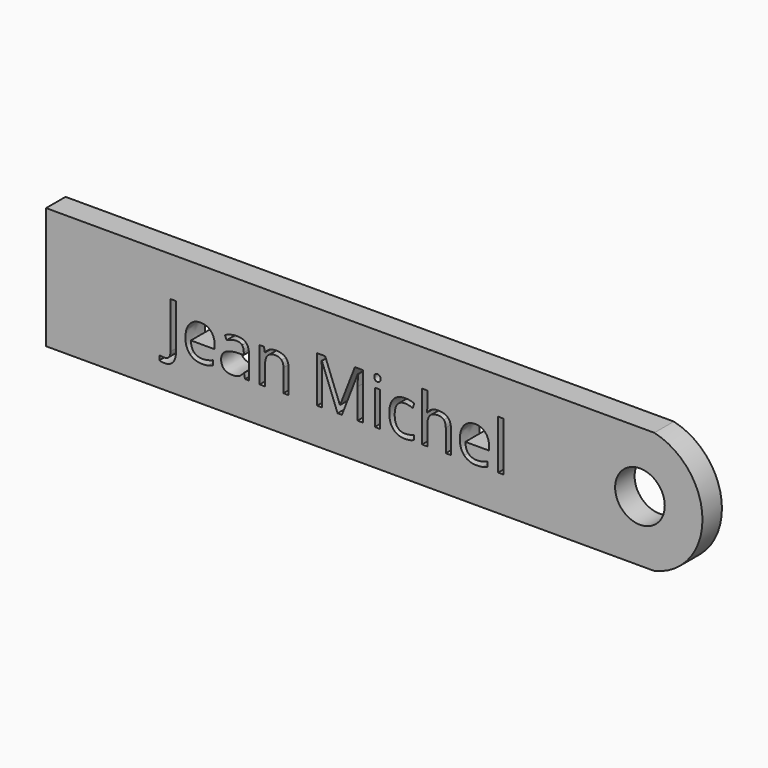
from build123d import *

# Parameters (mm, degrees)
F0_W     = 0.4318458111
F0_H     = 2.8498495239
F0_H_2   = 4.0463702874
F0_R     = 2.0408732003
F1_DEPTH = 2


with BuildPart() as f1:
    # F0 (on Front) → F1 (new body)
    with BuildSketch(Plane.XZ):
        with BuildLine():
            Line((30.7838568464, 24.9683012729), (-19.2161431536, 24.9683012729))
            Line((-19.2161431536, 24.9683012729), (-19.2161431536, 14.9683012729))
            Line((-19.2161431536, 14.9683012729), (30.7838568464, 14.9683012729))
            ThreePointArc((30.7838568464, 14.9683012729), (34.7379549914, 19.9683012729), (30.7838568464, 24.9683012729))
        make_face()
        with BuildLine():
            add(Edge.make_bspline(
                [(-8.7974733445, 17.1836813513), (-9.0470952006, 16.9120095646), (-9.5155522172, 16.9120095646)],
                knots=[0, 0, 0, 1, 1, 1], degree=2))
            add(Edge.make_bspline(
                [(-9.5155522172, 16.9120095646), (-9.7593495634, 16.9120095646), (-9.8999698756, 16.9819036843)],
                knots=[0, 0, 0, 1, 1, 1], degree=2))
            Line((-9.8999698756, 16.9819036843), (-9.8999698756, 17.358832687))
            add(Edge.make_bspline(
                [(-9.8999698756, 17.358832687), (-9.7152497021, 17.3072441701), (-9.5155522172, 17.3072441701)],
                knots=[0, 0, 0, 1, 1, 1], degree=2))
            add(Edge.make_bspline(
                [(-9.5155522172, 17.3072441701), (-9.2576096326, 17.3072441701), (-9.1236459031, 17.4632578302)],
                knots=[0, 0, 0, 1, 1, 1], degree=2))
            add(Edge.make_bspline(
                [(-9.1236459031, 17.4632578302), (-8.9896821737, 17.6192714902), (-8.9896821737, 17.9129932076)],
                knots=[0, 0, 0, 1, 1, 1], degree=2))
            Line((-8.9896821737, 17.9129932076), (-8.9896821737, 21.714734076))
            Line((-8.9896821737, 21.714734076), (-8.5478514884, 21.714734076))
            Line((-8.5478514884, 21.714734076), (-8.5478514884, 17.9496044131))
            add(Edge.make_bspline(
                [(-8.5478514884, 17.9496044131), (-8.5478514884, 17.455353138), (-8.7974733445, 17.1836813513)],
                knots=[0, 0, 0, 1, 1, 1], degree=2))
        make_face(mode=Mode.SUBTRACT)
        with BuildLine():
            add(Edge.make_bspline(
                [(-5.9076843237, 17.9038404062), (-6.1115421728, 17.8605726178), (-6.4002714531, 17.8605726178)],
                knots=[0, 0, 0, 1, 1, 1], degree=2))
            add(Edge.make_bspline(
                [(-6.4002714531, 17.8605726178), (-7.031814749, 17.8605726178), (-7.3975107682, 18.245822349)],
                knots=[0, 0, 0, 1, 1, 1], degree=2))
            add(Edge.make_bspline(
                [(-7.3975107682, 18.245822349), (-7.7632067874, 18.6310720803), (-7.7632067874, 19.3142038932)],
                knots=[0, 0, 0, 1, 1, 1], degree=2))
            add(Edge.make_bspline(
                [(-7.7632067874, 19.3142038932), (-7.7632067874, 20.0039922889), (-7.4237210631, 20.409627805)],
                knots=[0, 0, 0, 1, 1, 1], degree=2))
            add(Edge.make_bspline(
                [(-7.4237210631, 20.409627805), (-7.0842353388, 20.8152633212), (-6.5117692154, 20.8152633212)],
                knots=[0, 0, 0, 1, 1, 1], degree=2))
            add(Edge.make_bspline(
                [(-6.5117692154, 20.8152633212), (-5.9767463705, 20.8152633212), (-5.6647190504, 20.4628804677)],
                knots=[0, 0, 0, 1, 1, 1], degree=2))
            add(Edge.make_bspline(
                [(-5.6647190504, 20.4628804677), (-5.3526917303, 20.1104976141), (-5.3526917303, 19.5330390537)],
                knots=[0, 0, 0, 1, 1, 1], degree=2))
            Line((-5.3526917303, 19.5330390537), (-5.3526917303, 19.2601191577))
            Line((-5.3526917303, 19.2601191577), (-7.3155515921, 19.2601191577))
            add(Edge.make_bspline(
                [(-7.3155515921, 19.2601191577), (-7.3022384264, 18.7583792269), (-7.0617693717, 18.4983564601)],
                knots=[0, 0, 0, 1, 1, 1], degree=2))
            add(Edge.make_bspline(
                [(-7.0617693717, 18.4983564601), (-6.821300317, 18.2383336934), (-6.3844620688, 18.2383336934)],
                knots=[0, 0, 0, 1, 1, 1], degree=2))
            add(Edge.make_bspline(
                [(-6.3844620688, 18.2383336934), (-5.9243257807, 18.2383336934), (-5.4750064398, 18.4305425226)],
                knots=[0, 0, 0, 1, 1, 1], degree=2))
            Line((-5.4750064398, 18.4305425226), (-5.4750064398, 18.0452927913))
            add(Edge.make_bspline(
                [(-5.4750064398, 18.0452927913), (-5.7038264745, 17.9471081946), (-5.9076843237, 17.9038404062)],
                knots=[0, 0, 0, 1, 1, 1], degree=2))
        make_face(mode=Mode.SUBTRACT)
        with BuildLine():
            Line((-2.5436137762, 17.9129932076), (-2.8639618249, 17.9129932076))
            Line((-2.8639618249, 17.9129932076), (-2.9496653288, 18.3190447602))
            Line((-2.9496653288, 18.3190447602), (-2.9704671502, 18.3190447602))
            add(Edge.make_bspline(
                [(-2.9704671502, 18.3190447602), (-3.1834778007, 18.0511173013), (-3.395240342, 17.9558449595)],
                knots=[0, 0, 0, 1, 1, 1], degree=2))
            add(Edge.make_bspline(
                [(-3.395240342, 17.9558449595), (-3.6070028833, 17.8605726178), (-3.9248547134, 17.8605726178)],
                knots=[0, 0, 0, 1, 1, 1], degree=2))
            add(Edge.make_bspline(
                [(-3.9248547134, 17.8605726178), (-4.3483797959, 17.8605726178), (-4.5888488506, 18.0794077783)],
                knots=[0, 0, 0, 1, 1, 1], degree=2))
            add(Edge.make_bspline(
                [(-4.5888488506, 18.0794077783), (-4.8293179053, 18.2982429388), (-4.8293179053, 18.7009662)],
                knots=[0, 0, 0, 1, 1, 1], degree=2))
            add(Edge.make_bspline(
                [(-4.8293179053, 18.7009662), (-4.8293179053, 19.5638257493), (-3.4489090411, 19.605429392)],
                knots=[0, 0, 0, 1, 1, 1], degree=2))
            Line((-3.4489090411, 19.605429392), (-2.9654747131, 19.6212387762))
            Line((-2.9654747131, 19.6212387762), (-2.9654747131, 19.798470294))
            add(Edge.make_bspline(
                [(-2.9654747131, 19.798470294), (-2.9654747131, 20.133795654), (-3.1094233168, 20.293553642)],
                knots=[0, 0, 0, 1, 1, 1], degree=2))
            add(Edge.make_bspline(
                [(-3.1094233168, 20.293553642), (-3.2533719204, 20.4533116299), (-3.5712237505, 20.4533116299)],
                knots=[0, 0, 0, 1, 1, 1], degree=2))
            add(Edge.make_bspline(
                [(-3.5712237505, 20.4533116299), (-3.9273509319, 20.4533116299), (-4.3766702729, 20.2353085422)],
                knots=[0, 0, 0, 1, 1, 1], degree=2))
            Line((-4.3766702729, 20.2353085422), (-4.5098019295, 20.5656414651))
            add(Edge.make_bspline(
                [(-4.5098019295, 20.5656414651), (-4.2992874975, 20.6796354461), (-4.0484175321, 20.7445371286)],
                knots=[0, 0, 0, 1, 1, 1], degree=2))
            add(Edge.make_bspline(
                [(-4.0484175321, 20.7445371286), (-3.7975475667, 20.8094388112), (-3.5445974192, 20.8094388112)],
                knots=[0, 0, 0, 1, 1, 1], degree=2))
            add(Edge.make_bspline(
                [(-3.5445974192, 20.8094388112), (-3.0353688328, 20.8094388112), (-2.7894913045, 20.5835310315)],
                knots=[0, 0, 0, 1, 1, 1], degree=2))
            add(Edge.make_bspline(
                [(-2.7894913045, 20.5835310315), (-2.5436137762, 20.3576232517), (-2.5436137762, 19.8583795395)],
                knots=[0, 0, 0, 1, 1, 1], degree=2))
            Line((-2.5436137762, 19.8583795395), (-2.5436137762, 17.9129932076))
        make_face(mode=Mode.SUBTRACT)
        with BuildLine():
            Line((0.7272646116, 17.9129932076), (0.2954188005, 17.9129932076))
            Line((0.2954188005, 17.9129932076), (0.2954188005, 19.7568666513))
            add(Edge.make_bspline(
                [(0.2954188005, 19.7568666513), (0.2954188005, 20.1046731042), (0.1369089219, 20.2764961485)],
                knots=[0, 0, 0, 1, 1, 1], degree=2))
            add(Edge.make_bspline(
                [(0.1369089219, 20.2764961485), (-0.0216009567, 20.4483191927), (-0.3602546082, 20.4483191927)],
                knots=[0, 0, 0, 1, 1, 1], degree=2))
            add(Edge.make_bspline(
                [(-0.3602546082, 20.4483191927), (-0.8070777306, 20.4483191927), (-1.015095944, 20.2066020287)],
                knots=[0, 0, 0, 1, 1, 1], degree=2))
            add(Edge.make_bspline(
                [(-1.015095944, 20.2066020287), (-1.2231141575, 19.9648848647), (-1.2231141575, 19.4082281256)],
                knots=[0, 0, 0, 1, 1, 1], degree=2))
            Line((-1.2231141575, 19.4082281256), (-1.2231141575, 17.9129932076))
            Line((-1.2231141575, 17.9129932076), (-1.6549599685, 17.9129932076))
            Line((-1.6549599685, 17.9129932076), (-1.6549599685, 20.7628427314))
            Line((-1.6549599685, 20.7628427314), (-1.3038252243, 20.7628427314))
            Line((-1.3038252243, 20.7628427314), (-1.2339311046, 20.3726005631))
            Line((-1.2339311046, 20.3726005631), (-1.2131292832, 20.3726005631))
            add(Edge.make_bspline(
                [(-1.2131292832, 20.3726005631), (-1.0799976266, 20.583114995), (-0.8407766812, 20.6991891581)],
                knots=[0, 0, 0, 1, 1, 1], degree=2))
            add(Edge.make_bspline(
                [(-0.8407766812, 20.6991891581), (-0.6015557358, 20.8152633212), (-0.3078340184, 20.8152633212)],
                knots=[0, 0, 0, 1, 1, 1], degree=2))
            add(Edge.make_bspline(
                [(-0.3078340184, 20.8152633212), (0.207219078, 20.8152633212), (0.4672418448, 20.5668895744)],
                knots=[0, 0, 0, 1, 1, 1], degree=2))
            add(Edge.make_bspline(
                [(0.4672418448, 20.5668895744), (0.7272646116, 20.3185158276), (0.7272646116, 19.7718439627)],
                knots=[0, 0, 0, 1, 1, 1], degree=2))
            Line((0.7272646116, 19.7718439627), (0.7272646116, 17.9129932076))
        make_face(mode=Mode.SUBTRACT)
        with BuildLine():
            Line((5.1006395305, 17.9129932076), (4.7445123491, 17.9129932076))
            Line((4.7445123491, 17.9129932076), (3.4547994259, 21.282888265))
            Line((3.4547994259, 21.282888265), (3.4339976046, 21.282888265))
            add(Edge.make_bspline(
                [(3.4339976046, 21.282888265), (3.4706088102, 20.8826612224), (3.4706088102, 20.3309969204)],
                knots=[0, 0, 0, 1, 1, 1], degree=2))
            Line((3.4706088102, 20.3309969204), (3.4706088102, 17.9129932076))
            Line((3.4706088102, 17.9129932076), (3.062061039, 17.9129932076))
            Line((3.062061039, 17.9129932076), (3.062061039, 21.714734076))
            Line((3.062061039, 21.714734076), (3.7277193219, 21.714734076))
            Line((3.7277193219, 21.714734076), (4.9317287412, 18.5786514905))
            Line((4.9317287412, 18.5786514905), (4.9525305626, 18.5786514905))
            Line((4.9525305626, 18.5786514905), (6.1665248561, 21.714734076))
            Line((6.1665248561, 21.714734076), (6.8271907019, 21.714734076))
            Line((6.8271907019, 21.714734076), (6.8271907019, 17.9129932076))
            Line((6.8271907019, 17.9129932076), (6.3853600166, 17.9129932076))
            Line((6.3853600166, 17.9129932076), (6.3853600166, 20.3626156888))
            add(Edge.make_bspline(
                [(6.3853600166, 20.3626156888), (6.3853600166, 20.7836445528), (6.4219712222, 21.2778958279)],
                knots=[0, 0, 0, 1, 1, 1], degree=2))
            Line((6.4219712222, 21.2778958279), (6.4011694008, 21.2778958279))
            Line((6.4011694008, 21.2778958279), (5.1006395305, 17.9129932076))
        make_face(mode=Mode.SUBTRACT)
        with Locations((8.0207992105, 19.3379179695)):
            Rectangle(F0_W, F0_H, mode=Mode.SUBTRACT)
        with BuildLine():
            add(Edge.make_bspline(
                [(11.0108530102, 18.0095136586), (10.7254520214, 17.8605726178), (10.2911099918, 17.8605726178)],
                knots=[0, 0, 0, 1, 1, 1], degree=2))
            add(Edge.make_bspline(
                [(10.2911099918, 17.8605726178), (9.6720477886, 17.8605726178), (9.3325620643, 18.2416619848)],
                knots=[0, 0, 0, 1, 1, 1], degree=2))
            add(Edge.make_bspline(
                [(9.3325620643, 18.2416619848), (8.99307634, 18.6227513518), (8.99307634, 19.3200284031)],
                knots=[0, 0, 0, 1, 1, 1], degree=2))
            add(Edge.make_bspline(
                [(8.99307634, 19.3200284031), (8.99307634, 20.0347789845), (9.3379705379, 20.4250211528)],
                knots=[0, 0, 0, 1, 1, 1], degree=2))
            add(Edge.make_bspline(
                [(9.3379705379, 20.4250211528), (9.6828647357, 20.8152633212), (10.3194004688, 20.8152633212)],
                knots=[0, 0, 0, 1, 1, 1], degree=2))
            add(Edge.make_bspline(
                [(10.3194004688, 20.8152633212), (10.5249224636, 20.8152633212), (10.7304444585, 20.7707474235)],
                knots=[0, 0, 0, 1, 1, 1], degree=2))
            add(Edge.make_bspline(
                [(10.7304444585, 20.7707474235), (10.9359664534, 20.7262315259), (11.0524566529, 20.6663222804)],
                knots=[0, 0, 0, 1, 1, 1], degree=2))
            Line((11.0524566529, 20.6663222804), (10.9201570691, 20.3002102248))
            add(Edge.make_bspline(
                [(10.9201570691, 20.3002102248), (10.7770405383, 20.3576232517), (10.608129749, 20.3950665301)],
                knots=[0, 0, 0, 1, 1, 1], degree=2))
            add(Edge.make_bspline(
                [(10.608129749, 20.3950665301), (10.4392189597, 20.4325098085), (10.3094155945, 20.4325098085)],
                knots=[0, 0, 0, 1, 1, 1], degree=2))
            add(Edge.make_bspline(
                [(10.3094155945, 20.4325098085), (9.4407315353, 20.4325098085), (9.4407315353, 19.3250208403)],
                knots=[0, 0, 0, 1, 1, 1], degree=2))
            add(Edge.make_bspline(
                [(9.4407315353, 19.3250208403), (9.4407315353, 18.7999828696), (9.6524940766, 18.5191582815)],
                knots=[0, 0, 0, 1, 1, 1], degree=2))
            add(Edge.make_bspline(
                [(9.6524940766, 18.5191582815), (9.8642566178, 18.2383336934), (10.2802930447, 18.2383336934)],
                knots=[0, 0, 0, 1, 1, 1], degree=2))
            add(Edge.make_bspline(
                [(10.2802930447, 18.2383336934), (10.636420226, 18.2383336934), (11.0108530102, 18.3914350984)],
                knots=[0, 0, 0, 1, 1, 1], degree=2))
            Line((11.0108530102, 18.3914350984), (11.0108530102, 18.0095136586))
        make_face(mode=Mode.SUBTRACT)
        with BuildLine():
            Line((14.0695528203, 17.9129932076), (13.6377070093, 17.9129932076))
            Line((13.6377070093, 17.9129932076), (13.6377070093, 19.7568666513))
            add(Edge.make_bspline(
                [(13.6377070093, 19.7568666513), (13.6377070093, 20.1046731042), (13.4791971306, 20.2764961485)],
                knots=[0, 0, 0, 1, 1, 1], degree=2))
            add(Edge.make_bspline(
                [(13.4791971306, 20.2764961485), (13.320687252, 20.4483191927), (12.9820336006, 20.4483191927)],
                knots=[0, 0, 0, 1, 1, 1], degree=2))
            add(Edge.make_bspline(
                [(12.9820336006, 20.4483191927), (12.5327142596, 20.4483191927), (12.3259441554, 20.2036897738)],
                knots=[0, 0, 0, 1, 1, 1], degree=2))
            add(Edge.make_bspline(
                [(12.3259441554, 20.2036897738), (12.1191740513, 19.9590603548), (12.1191740513, 19.4032356885)],
                knots=[0, 0, 0, 1, 1, 1], degree=2))
            Line((12.1191740513, 19.4032356885), (12.1191740513, 17.9129932076))
            Line((12.1191740513, 17.9129932076), (11.6873282402, 17.9129932076))
            Line((11.6873282402, 17.9129932076), (11.6873282402, 21.959363495))
            Line((11.6873282402, 21.959363495), (12.1191740513, 21.959363495))
            Line((12.1191740513, 21.959363495), (12.1191740513, 20.7345522544))
            add(Edge.make_bspline(
                [(12.1191740513, 20.7345522544), (12.1191740513, 20.5132208753), (12.09837223, 20.3676081259)],
                knots=[0, 0, 0, 1, 1, 1], degree=2))
            Line((12.09837223, 20.3676081259), (12.1241664884, 20.3676081259))
            add(Edge.make_bspline(
                [(12.1241664884, 20.3676081259), (12.251473635, 20.5731301208), (12.4869502526, 20.691284466)],
                knots=[0, 0, 0, 1, 1, 1], degree=2))
            add(Edge.make_bspline(
                [(12.4869502526, 20.691284466), (12.7224268702, 20.8094388112), (13.0236372432, 20.8094388112)],
                knots=[0, 0, 0, 1, 1, 1], degree=2))
            add(Edge.make_bspline(
                [(13.0236372432, 20.8094388112), (13.5461789954, 20.8094388112), (13.8078659078, 20.5610650644)],
                knots=[0, 0, 0, 1, 1, 1], degree=2))
            add(Edge.make_bspline(
                [(13.8078659078, 20.5610650644), (14.0695528203, 20.3126913176), (14.0695528203, 19.7718439627)],
                knots=[0, 0, 0, 1, 1, 1], degree=2))
            Line((14.0695528203, 19.7718439627), (14.0695528203, 17.9129932076))
        make_face(mode=Mode.SUBTRACT)
        with BuildLine():
            add(Edge.make_bspline(
                [(16.6523069581, 17.9038404062), (16.448449109, 17.8605726178), (16.1597198288, 17.8605726178)],
                knots=[0, 0, 0, 1, 1, 1], degree=2))
            add(Edge.make_bspline(
                [(16.1597198288, 17.8605726178), (15.5281765328, 17.8605726178), (15.1624805136, 18.245822349)],
                knots=[0, 0, 0, 1, 1, 1], degree=2))
            add(Edge.make_bspline(
                [(15.1624805136, 18.245822349), (14.7967844944, 18.6310720803), (14.7967844944, 19.3142038932)],
                knots=[0, 0, 0, 1, 1, 1], degree=2))
            add(Edge.make_bspline(
                [(14.7967844944, 19.3142038932), (14.7967844944, 20.0039922889), (15.1362702187, 20.409627805)],
                knots=[0, 0, 0, 1, 1, 1], degree=2))
            add(Edge.make_bspline(
                [(15.1362702187, 20.409627805), (15.475755943, 20.8152633212), (16.0482220664, 20.8152633212)],
                knots=[0, 0, 0, 1, 1, 1], degree=2))
            add(Edge.make_bspline(
                [(16.0482220664, 20.8152633212), (16.5832449113, 20.8152633212), (16.8952722314, 20.4628804677)],
                knots=[0, 0, 0, 1, 1, 1], degree=2))
            add(Edge.make_bspline(
                [(16.8952722314, 20.4628804677), (17.2072995516, 20.1104976141), (17.2072995516, 19.5330390537)],
                knots=[0, 0, 0, 1, 1, 1], degree=2))
            Line((17.2072995516, 19.5330390537), (17.2072995516, 19.2601191577))
            Line((17.2072995516, 19.2601191577), (15.2444396897, 19.2601191577))
            add(Edge.make_bspline(
                [(15.2444396897, 19.2601191577), (15.2577528554, 18.7583792269), (15.4982219101, 18.4983564601)],
                knots=[0, 0, 0, 1, 1, 1], degree=2))
            add(Edge.make_bspline(
                [(15.4982219101, 18.4983564601), (15.7386909648, 18.2383336934), (16.175529213, 18.2383336934)],
                knots=[0, 0, 0, 1, 1, 1], degree=2))
            add(Edge.make_bspline(
                [(16.175529213, 18.2383336934), (16.6356655011, 18.2383336934), (17.0849848421, 18.4305425226)],
                knots=[0, 0, 0, 1, 1, 1], degree=2))
            Line((17.0849848421, 18.4305425226), (17.0849848421, 18.0452927913))
            add(Edge.make_bspline(
                [(17.0849848421, 18.0452927913), (16.8561648073, 17.9471081946), (16.6523069581, 17.9038404062)],
                knots=[0, 0, 0, 1, 1, 1], degree=2))
        make_face(mode=Mode.SUBTRACT)
        with Locations((18.1596069326, 19.9361783513)):
            Rectangle(F0_W, F0_H_2, mode=Mode.SUBTRACT)
        with BuildLine():
            add(Edge.make_bspline(
                [(7.8410714741, 21.3178353248), (7.7682650994, 21.3893935902), (7.7682650994, 21.5350063396)],
                knots=[0, 0, 0, 1, 1, 1], degree=2))
            add(Edge.make_bspline(
                [(7.7682650994, 21.5350063396), (7.7682650994, 21.6831153076), (7.8410714741, 21.7521773545)],
                knots=[0, 0, 0, 1, 1, 1], degree=2))
            add(Edge.make_bspline(
                [(7.8410714741, 21.7521773545), (7.9138778488, 21.8212394013), (8.0237114655, 21.8212394013)],
                knots=[0, 0, 0, 1, 1, 1], degree=2))
            add(Edge.make_bspline(
                [(8.0237114655, 21.8212394013), (8.1277205722, 21.8212394013), (8.2030231655, 21.7509292452)],
                knots=[0, 0, 0, 1, 1, 1], degree=2))
            add(Edge.make_bspline(
                [(8.2030231655, 21.7509292452), (8.2783257587, 21.680619089), (8.2783257587, 21.5350063396)],
                knots=[0, 0, 0, 1, 1, 1], degree=2))
            add(Edge.make_bspline(
                [(8.2783257587, 21.5350063396), (8.2783257587, 21.3893935902), (8.2030231655, 21.3178353248)],
                knots=[0, 0, 0, 1, 1, 1], degree=2))
            add(Edge.make_bspline(
                [(8.2030231655, 21.3178353248), (8.1277205722, 21.2462770594), (8.0237114655, 21.2462770594)],
                knots=[0, 0, 0, 1, 1, 1], degree=2))
            add(Edge.make_bspline(
                [(8.0237114655, 21.2462770594), (7.9138778488, 21.2462770594), (7.8410714741, 21.3178353248)],
                knots=[0, 0, 0, 1, 1, 1], degree=2))
        make_face(mode=Mode.SUBTRACT)
        with Locations((29.5996287979, 19.9683012729)):
            Circle(F0_R, mode=Mode.SUBTRACT)
    extrude(amount=F1_DEPTH)


solid = f1.part
